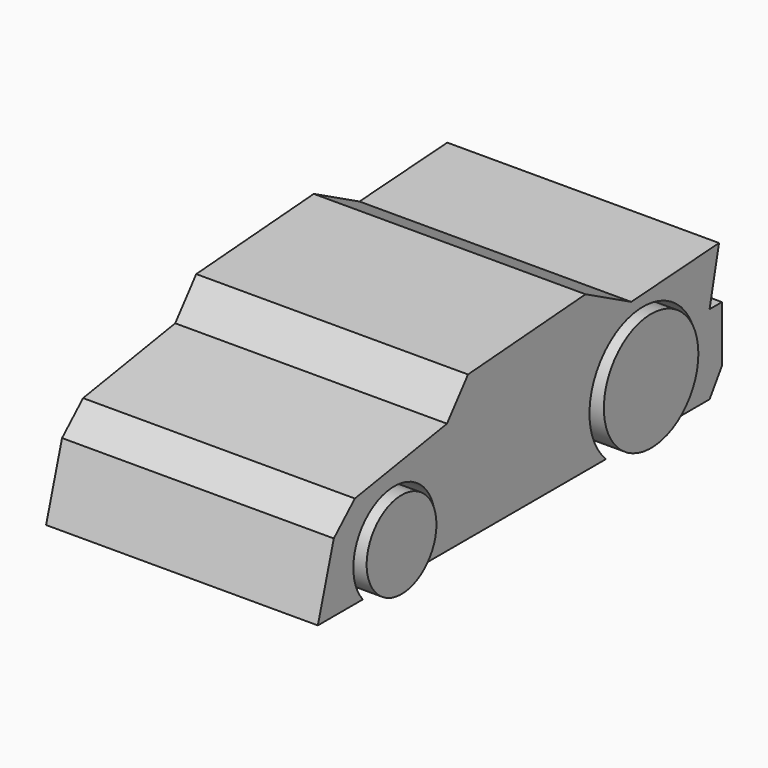
from build123d import *

# Parameters (mm, degrees)
F1_DEPTH      = 47.52499
F1_DEPTH_BACK = 29.45433
F2_R          = 14.4647105866
F2_R_2        = 18.9829948576
F3_DEPTH      = 83.41263
F3_DEPTH_BACK = 94.24229
F4_R          = 12.3503734922
F5_DEPTH      = 49.65811
F5_DEPTH_BACK = 30.90248
F4_R_2        = 16.7330051387


# Not quite as in the source:
# - a feature of the source that left no trace in its solid (it failed there, or was rolled back) is left out


with BuildPart() as f1:
    # F0 (on Right) → F1 (new body, two sides)
    with BuildSketch(Plane.YZ) as f1_sk:
        Polygon((-68.0662915111, 19.3924717605), (-73.7170800567, 0), (64.9840459228, 0), (69.3505629897, 6.5497751348), (69.3505629897, 22.4747192115), (64.9840459228, 22.4747192115), (68.3231502771, 37.6291014254), (37.2438170016, 35.5742685497), (21.0620239377, 44.0504476428), (-20.5483157188, 40.9682020545), (-27.997078374, 31.7214615643), (-60.6175288558, 26.3275280595), align=None)
    extrude(amount=F1_DEPTH)
    extrude(f1_sk.sketch, amount=-F1_DEPTH_BACK)

    # F2 (on Right) → F3 (cut, two sides)
    with BuildSketch(Plane.YZ) as f3_sk:
        with Locations((-46.6906875372, 9.2489616945)):
            Circle(F2_R)
        with Locations((41.4386764169, 13.7112075463)):
            Circle(F2_R_2)
    extrude(amount=F3_DEPTH, mode=Mode.SUBTRACT)
    extrude(f3_sk.sketch, amount=-F3_DEPTH_BACK, mode=Mode.SUBTRACT)


with BuildPart() as f5:
    # F4 (on Right) → F5 (new body, two sides)
    with BuildSketch(Plane.YZ) as f5_sk:
        with Locations((-46.7474162579, 9.8888762295)):
            Circle(F4_R)
    extrude(amount=F5_DEPTH)
    extrude(f5_sk.sketch, amount=-F5_DEPTH_BACK)


with BuildPart() as f5b:
    # F4 (on Right) → F5, piece 2 (new body, two sides)
    with BuildSketch(Plane.YZ) as f5_2_sk:
        with Locations((41.6103377938, 14.7691015154)):
            Circle(F4_R_2)
    extrude(amount=F5_DEPTH)
    extrude(f5_2_sk.sketch, amount=-F5_DEPTH_BACK)


solid = Compound([f1.part, f5.part, f5b.part])
